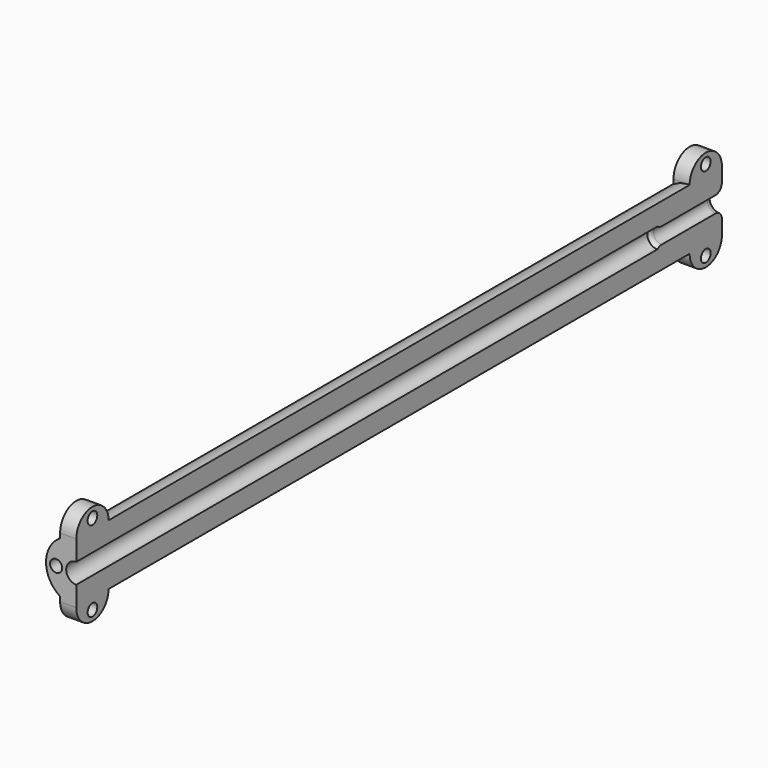
from build123d import *

# Parameters (mm, degrees)
F0_R         = 7.5
F0_R_2       = 2.5
F1_DEPTH     = 200
F2_R         = 1.5
F3_DEPTH     = 25
F4_W         = 255.6320726871
F4_H         = 34.7503256053
F5_DEPTH     = 25
F6_W         = 10
F6_H         = 5
F6_H_2       = 4.8793365061
F7_DEPTH     = 4
F8_R         = 1.5
F9_DEPTH     = 7.501
F11_DEPTH    = 20
F12_T2_ANGLE = 359.64
F12_T4_ANGLE = 359.64


# Not quite as in the source:
# - a fillet or chamfer that OpenCascade refuses, or shapes differently, is made with other operations: its cross-section is extruded or revolved along the edge and cut away or added


with BuildPart() as f1:
    # F0 (on Front) → F1 (new body)
    with BuildSketch(Plane.XZ):
        Circle(F0_R)
        Circle(F0_R_2, mode=Mode.SUBTRACT)
    extrude(amount=-F1_DEPTH)

    # F2 (on face) → F3 (cut)
    with BuildSketch(Plane.XZ):
        with Locations((5, 0)):
            Circle(F2_R)
        with Locations((-5, 0)):
            Circle(F2_R)
    extrude(amount=-F3_DEPTH, mode=Mode.SUBTRACT)

    # F4 (on Right) → F5 (cut)
    with BuildSketch(Plane.YZ):
        with Locations((127.8160363436, -0.9753750637)):
            Rectangle(F4_W, F4_H)
    extrude(amount=F5_DEPTH, mode=Mode.SUBTRACT)

    # F6 (on face) → F7 (join)
    with BuildSketch(Plane.YZ):
        with BuildLine():
            ThreePointArc((10, 7.5), (5, 12.5), (0, 7.5))
            Line((0, 7.5), (10, 7.5))
        make_face()
        with Locations((5, 5)):
            Rectangle(F6_W, F6_H)
        with BuildLine():
            Line((190, 7.5), (200, 7.5))
            ThreePointArc((200, 7.5), (195, 12.5), (190, 7.5))
        make_face()
        with Locations((195, 5)):
            Rectangle(F6_W, F6_H)
        with BuildLine():
            ThreePointArc((190, -7.5), (195, -12.5), (200, -7.5))
            Line((200, -7.5), (190, -7.5))
        make_face()
        with Locations((195, -5.0603317469)):
            Rectangle(F6_W, F6_H_2)
        with BuildLine():
            Line((10, -7.5), (0, -7.5))
            ThreePointArc((0, -7.5), (5, -12.5), (10, -7.5))
        make_face()
        with Locations((5, -5.0603317469)):
            Rectangle(F6_W, F6_H_2)
    extrude(amount=-F7_DEPTH)

    # F8 (on face) → F9 (cut, through all)
    with BuildSketch(Plane.YZ):
        with Locations((5, 10)):
            Circle(F8_R)
        with Locations((5, -10)):
            Circle(F8_R)
        with Locations((195, 10)):
            Circle(F8_R)
        with Locations((195, -10)):
            Circle(F8_R)
    extrude(amount=-F9_DEPTH, mode=Mode.SUBTRACT)

    # F10 (on face) → F11 (join)
    with BuildSketch(Plane(origin=(0, 200, 0), x_dir=(-1, 0, 0), z_dir=(0, 1, 0))):
        with BuildLine():
            ThreePointArc((0, 2), (2, 0), (0, -2))
            Line((0, -2), (0, -2.5))
            ThreePointArc((0, -2.5), (2.5, 0), (0, 2.5))
            Line((0, 2.5), (0, 2))
        make_face()
    extrude(amount=-F11_DEPTH)

    # F12: fillet of radius 2 on 2 edges, made by hand

    # F12_s1 → F12_t2 (revolve, cut)
    with BuildSketch(Plane(origin=(0, 0, 0), x_dir=(0, 1, 0), z_dir=(0.0031415875, 0, -0.9999950652))):
        with BuildLine():
            ThreePointArc((180, 2.5), (180.6157688743, 2.1291713066), (181.3228756555, 2))
            Line((181.3228756555, 2), (180, 2))
            Line((180, 2), (180, 2.5))
        make_face()
    revolve(axis=Axis((0, 180, 0), (0, -1, 0)), revolution_arc=F12_T2_ANGLE, mode=Mode.SUBTRACT)

    # F12_s3 → F12_t4 (revolve, cut)
    with BuildSketch(Plane(origin=(0, 0, 0), x_dir=(0, 1, 0), z_dir=(0.0031415875, 0, -0.9999950652))):
        with BuildLine():
            ThreePointArc((198, 2), (199.4142135624, 2.5857864376), (200, 4))
            Line((200, 4), (200, 2))
            Line((200, 2), (198, 2))
        make_face()
    revolve(axis=Axis((0, 200, 0), (0, -1, 0)), revolution_arc=F12_T4_ANGLE, mode=Mode.SUBTRACT)


solid = f1.part
